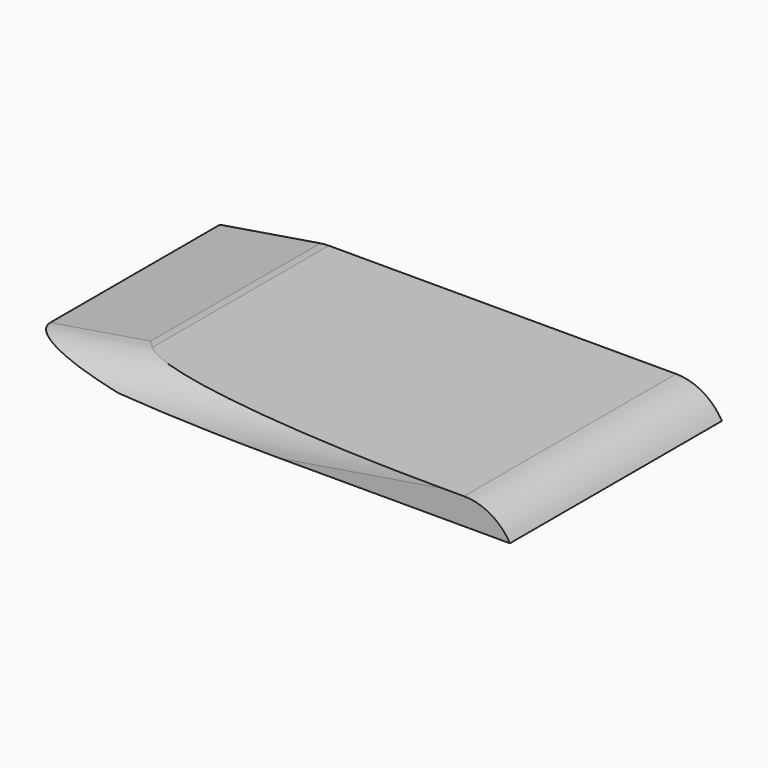
from build123d import *

# Parameters (mm, degrees)
F1_DEPTH    = 25.4
F2_T1_DEPTH = 60.96
F2_T3_DEPTH = 27.4503028349
F2_T5_DEPTH = 47.3970452561


# Not quite as in the source:
# - a fillet or chamfer that OpenCascade refuses, or shapes differently, is made with other operations: its cross-section is extruded or revolved along the edge and cut away or added


with BuildPart() as f1:
    # F0 (on Front) → F1 (new body)
    with BuildSketch(Plane.XZ):
        Polygon((-7.7007450502, 1.6296239436), (-17.7292008537, 0), (-7.7007450502, -0.9103760564), (30.3992549498, -0.9103760564), (30.3992549498, 1.6296239436), align=None)
    extrude(amount=F1_DEPTH)

    # F2: fillet of radius 5.08 on 3 edges, made by hand

    # F2_s2 → F2_t1 (cut)
    with BuildSketch(Plane(origin=(30.3620815059, 0, 4.9338378678), x_dir=(0, 1, 0), z_dir=(-0.9870527366, 0, -0.1603960574))):
        with BuildLine():
            ThreePointArc((-20.32, -2.8436939185), (-23.9121024484, -1.3557963669), (-25.4, 2.2363060815))
            Line((-25.4, 2.2363060815), (-25.4, -2.8436939185))
            Line((-25.4, -2.8436939185), (-20.32, -2.8436939185))
        make_face()
    extrude(amount=F2_T1_DEPTH, mode=Mode.SUBTRACT)

    # F2_s4 → F2_t3 (cut)
    with BuildSketch(Plane.XZ.offset(-1.0251514175)):
        with BuildLine():
            ThreePointArc((-7.2906844832, 1.6296239436), (-7.6994156046, 1.613154221), (-8.105496455, 1.5638518453))
            Line((-8.105496455, 1.5638518453), (-7.7007450502, 1.6296239436))
            Line((-7.7007450502, 1.6296239436), (-7.2906844832, 1.6296239436))
        make_face()
    extrude(amount=F2_T3_DEPTH, mode=Mode.SUBTRACT)

    # F2_s6 → F2_t5 (cut)
    with BuildSketch(Plane.XZ.offset(-10.9985226281)):
        with BuildLine():
            ThreePointArc((30.3992549498, -0.9103760564), (28.5398458985, 0.9490329948), (25.9998458985, 1.6296239436))
            Line((25.9998458985, 1.6296239436), (30.3992549498, 1.6296239436))
            Line((30.3992549498, 1.6296239436), (30.3992549498, -0.9103760564))
        make_face()
    extrude(amount=F2_T5_DEPTH, mode=Mode.SUBTRACT)


solid = f1.part
